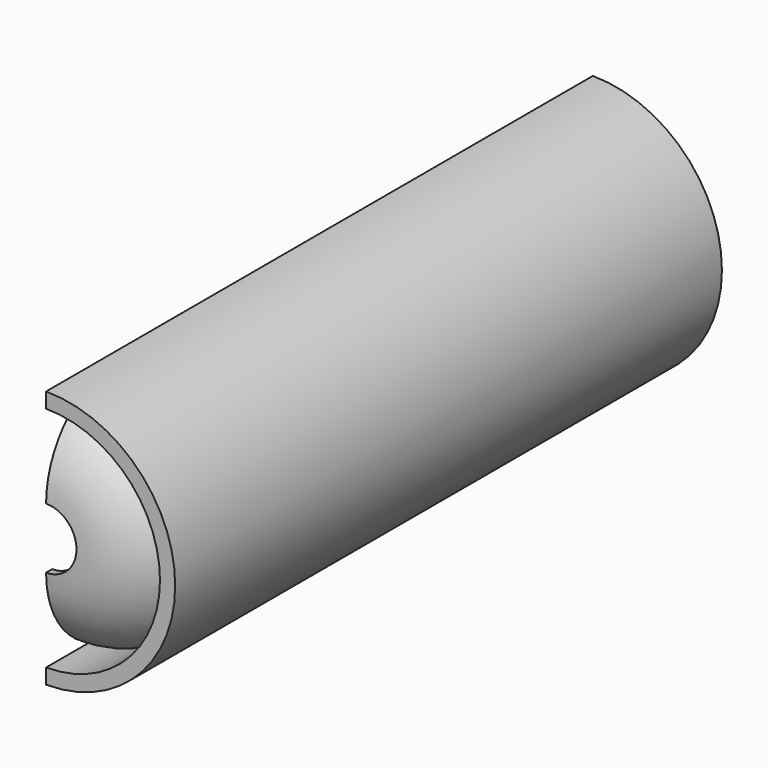
from build123d import *

# Parameters (mm, degrees)
F1_ANGLE = 180
F3_ANGLE = 180
F5_ANGLE = 180


# Not quite as in the source:
# - a feature names something its author has since deleted; it is built from what else it names


with BuildPart() as f1:
    # F0 (on Right) → F1 (revolve)
    with BuildSketch(Plane.YZ):
        with BuildLine():
            Line((86.8716222048, 34.384835436), (-3.1283777952, 34.384835436))
            Line((-3.1283777952, 34.384835436), (-3.1283777952, 32.384835436))
            Line((-3.1283777952, 32.384835436), (4.0757906815, 32.384835436))
            ThreePointArc((4.0757906815, 32.384835436), (-1.1670524657, 27.9594084914), (-3.1283777952, 21.384835436))
            Line((-3.1283777952, 21.384835436), (-2.1283777952, 21.384835436))
            ThreePointArc((-2.1283777952, 21.384835436), (1.0934476117, 29.1630100291), (8.8716222048, 32.384835436))
            Line((8.8716222048, 32.384835436), (71.8716222048, 32.384835436))
            ThreePointArc((71.8716222048, 32.384835436), (79.3046565784, 29.0966848666), (81.8716222048, 21.384835436))
            Line((81.8716222048, 21.384835436), (83.8716222048, 21.384835436))
            Line((83.8716222048, 21.384835436), (86.8716222048, 23.384835436))
            Line((86.8716222048, 23.384835436), (86.8716222048, 25.384835436))
            Line((86.8716222048, 25.384835436), (85.8716222048, 25.384835436))
            Line((85.8716222048, 25.384835436), (85.8716222048, 23.9200191945))
            Line((85.8716222048, 23.9200191945), (83.568846567, 22.384835436))
            Line((83.568846567, 22.384835436), (83.308739016, 22.384835436))
            ThreePointArc((83.308739016, 22.384835436), (82.1246676761, 28.0320507224), (78.337012641, 32.384835436))
            Line((78.337012641, 32.384835436), (86.8716222048, 32.384835436))
            Line((86.8716222048, 32.384835436), (86.8716222048, 34.384835436))
        make_face()
    revolve(axis=Axis((0, 40.3716222048, 17.384835436), (0, 1, 0)), revolution_arc=F1_ANGLE)


with BuildPart() as f3:
    # F2 (on Right) → F3 (revolve)
    with BuildSketch(Plane.YZ):
        with BuildLine():
            ThreePointArc((26.5840469152, 31.2761664331), (27.5840469152, 31.5441156255), (28.3160977227, 32.2761664331))
            Line((28.3160977227, 32.2761664331), (7.3641507709, 32.2761664331))
            ThreePointArc((7.3641507709, 32.2761664331), (1.3274941354, 29.3690617963), (-1.8600750098, 23.4756855441))
            Line((-1.8600750098, 23.4756855441), (-0.3631143027, 23.385647569))
            ThreePointArc((-0.3631143027, 23.385647569), (2.7686641904, 29.0327619647), (8.8238333804, 31.2761664331))
            Line((8.8238333804, 31.2761664331), (26.5840469152, 31.2761664331))
        make_face()
    revolve(axis=Axis((0, 40.3716222048, 17.384835436), (0, 1, 0)), revolution_arc=F3_ANGLE)


with BuildPart() as f5:
    # F4 (on Right) → F5 (revolve)
    with BuildSketch(Plane.YZ):
        Polygon((86.8716222048, 17.384835436), (86.8716222048, 22.7839102235), (84.0230100236, 20.884835436), (81.3716222048, 20.884835436), (81.3716222048, 20.384835436), (66.8716222048, 20.384835436), (66.8716222048, 17.384835436), (71.8716222048, 17.384835436), align=None)
    revolve(axis=Axis((0, 40.3716222048, 17.384835436), (0, 1, 0)), revolution_arc=F5_ANGLE)


solid = Compound([f1.part, f3.part, f5.part])
